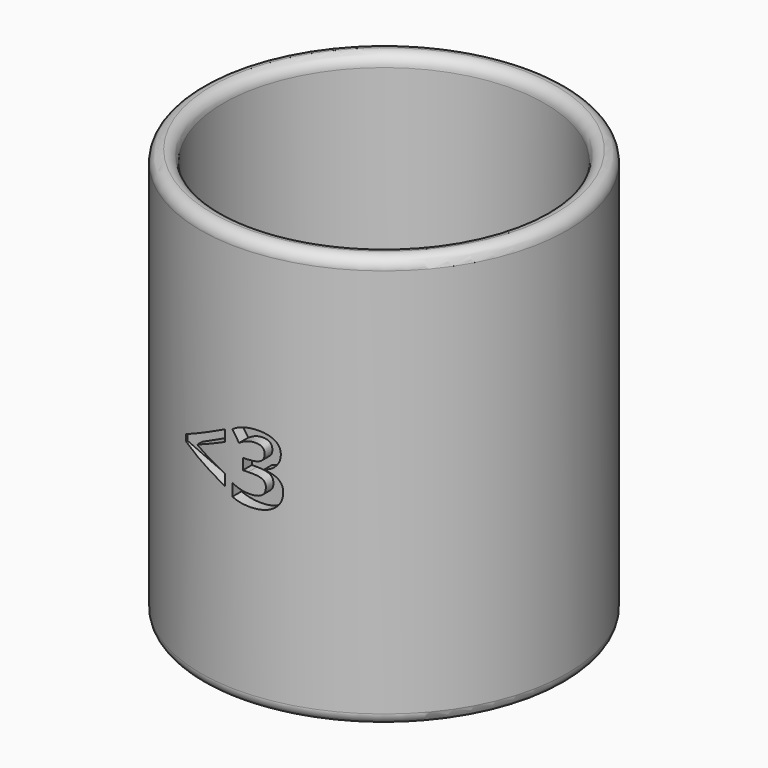
from build123d import *

# Parameters (mm, degrees)
F0_R          = 40
F1_DEPTH      = 90
F2_T          = -5
F7_R          = 2.49999
F8_TEXT_SIZE  = 25.7352962055
F9_DEPTH      = 1.75
F11_TEXT_SIZE = 20.7137782127
F12_DEPTH     = 2.5


# Not quite as in the source:
# - a fillet or chamfer is up to 0.001 mm smaller than in the source, because OpenCascade refuses the exact size
# - the program builds the solid bodies; features that only make, move or delete a surface that nothing else refers to are left out
# - Text() gives the source's letters only with a copy of the font that has no kerning and outlines rounded to 1/6400 em; it was checked with that copy


with BuildPart() as f1:
    # F0 (on Top) → F1 (new body)
    with BuildSketch(Plane.XY):
        Circle(F0_R)
    extrude(amount=F1_DEPTH)

    # F2
    f2_openings = [f1.faces().sort_by_distance(p)[0] for p in [
        (0, 0, 90),
    ]]
    offset(amount=F2_T, openings=f2_openings)

    # F7 (radius 2.5 in the source; OpenCascade refuses exactly that, so slightly less here)
    f7_edges = [f1.edges().sort_by_distance(p)[0] for p in [
        (-40, 0, 90),
        (-35, 0, 90),
        (-40, 0, 0),
    ]]
    fillet(f7_edges, radius=F7_R)

    # F8 (on face) → F9 (cut)
    with BuildSketch(Plane(origin=(0, 0, 0), x_dir=(1, 0, 0), z_dir=(0, 0, -1))):
        with Locations((-21.467000246, -8.2478486001)):
            Text('Boi', F8_TEXT_SIZE, font='Open Sans', font_style=FontStyle.BOLDITALIC, text_align=(TextAlign.LEFT, TextAlign.BOTTOM))
    extrude(amount=-F9_DEPTH, mode=Mode.SUBTRACT)

    # F11 (on offset) → F12 (cut)
    with BuildSketch(Plane.XZ.offset(40)):
        with Locations((-13.6710908264, 38.6949442327)):
            Text('<3', F11_TEXT_SIZE, font='Open Sans', font_style=FontStyle.BOLD, text_align=(TextAlign.LEFT, TextAlign.BOTTOM))
    extrude(amount=-F12_DEPTH, mode=Mode.SUBTRACT)


solid = f1.part
